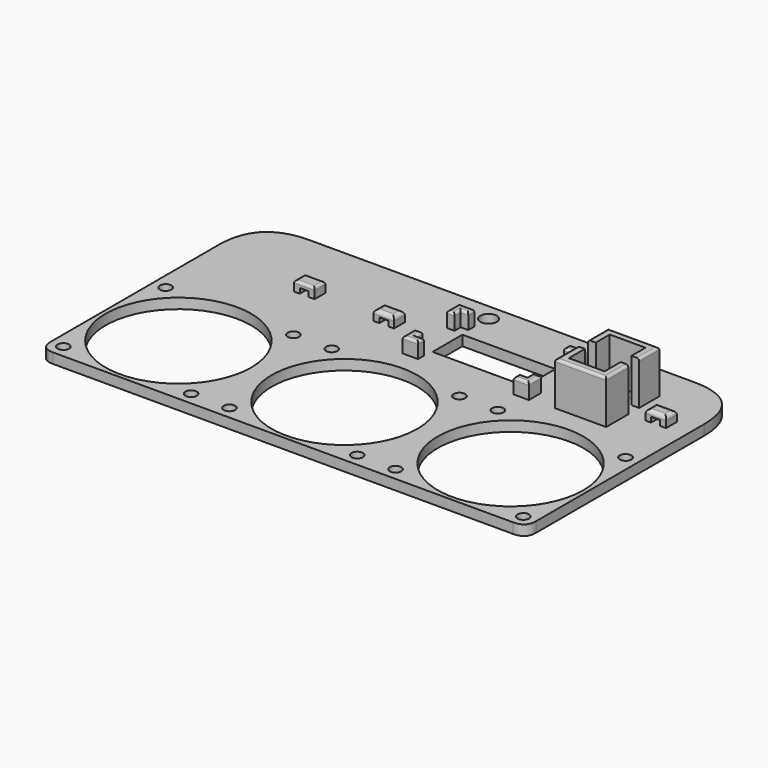
from build123d import *

# Parameters (mm, degrees)
F0_R         = 28.5
F1_DEPTH     = 4
F2_D         = 6.5
F3_D         = 4.5
F5_DEPTH     = 17
F6_DEPTH     = 6
F4_W         = 36.4
F4_H         = 14.6
F7_DEPTH     = 25
F4_W_2       = 7
F4_H_2       = 13
F8_DEPTH     = 25
F9_T1_DEPTH  = 104
F10_T1_DEPTH = 29
F4_W_3       = 8
F4_H_3       = 5.3025707603
F4_H_4       = 5.3
F11_DEPTH    = 4
F12_W        = 3.5351514816
F12_H        = 2
F13_DEPTH    = 25
F14_R        = 1.5
F15_R        = 1
F16_W        = 3.5
F16_H        = 2
F17_DEPTH    = 25
F18_R        = 1.5
F19_W        = 3.5
F19_H        = 2
F20_DEPTH    = 25
F21_R        = 1
F22_R        = 1


# Not quite as in the source:
# - a fillet or chamfer that OpenCascade refuses, or shapes differently, is made with other operations: its cross-section is extruded or revolved along the edge and cut away or added


with BuildPart() as f1:
    # F0 (on Top) → F1 (new body)
    with BuildSketch(Plane.XY):
        Polygon((0, 60), (0, 0), (60, 0), (65, 0), (125, 0), (130, 0), (190, 0), (190, 60), (190, 107), (0, 107), align=None)
        with Locations((30, 30)):
            Circle(F0_R, mode=Mode.SUBTRACT)
        with Locations((95, 30)):
            Circle(F0_R, mode=Mode.SUBTRACT)
        with Locations((160, 30)):
            Circle(F0_R, mode=Mode.SUBTRACT)
    extrude(amount=F1_DEPTH)

    # F2 (through all)
    with Locations(Plane(origin=(0, 0, 0), x_dir=(1, 0, 0), z_dir=(0, 0, -1))):
        with Locations((95, -100.5)):
            Hole(F2_D / 2)

    # F3 (through all)
    with Locations(Plane(origin=(0, 0, 0), x_dir=(1, 0, 0), z_dir=(0, 0, -1))):
        with Locations((5, -55), (55, -55), (5, -5), (55, -5), (70, -55), (70, -5), (120, -5), (120, -55), (135, -55), (135, -5), (185, -5), (185, -55)):
            Hole(F3_D / 2)

    # F4 (on face) → F5 (join)
    with BuildSketch(Plane.XY.offset(4)):
        Polygon((150.7997452021, 83.1751078367), (150.7997452021, 90), (164.7997452021, 90), (164.7997452021, 83.1751078367), (167.7997452021, 83.1751078367), (167.7997452021, 93), (147.7997452021, 93), (147.7997452021, 83.1751078367), align=None)
        Polygon((150.7997452021, 70), (150.7997452021, 77.8725370765), (147.7997452021, 77.8725370765), (147.7997452021, 67), (167.7997452021, 67), (167.7997452021, 77.8725370765), (164.7997452021, 77.8725370765), (164.7997452021, 70), align=None)
    extrude(amount=F5_DEPTH)

    # F4 (on face) → F6 (join)
    with BuildSketch(Plane.XY.offset(4)):
        Polygon((132.2073462009, 93.8), (132.2073462009, 90.8), (135.2073462009, 90.8), (135.2073462009, 87.8), (138.2073462009, 87.8), (138.2073462009, 93.8), align=None)
        Polygon((138.2073462009, 66.2), (138.2073462009, 72.2), (135.2073462009, 72.2), (135.2073462009, 69.2), (132.2073462009, 69.2), (132.2073462009, 66.2), align=None)
        Polygon((88.8073462009, 66.2), (94.8073462009, 66.2), (94.8073462009, 69.2), (91.8073462009, 69.2), (91.8073462009, 72.2), (88.8073462009, 72.2), align=None)
        Polygon((88.8073462009, 87.8), (91.8073462009, 87.8), (91.8073462009, 90.8), (94.8073462009, 90.8), (94.8073462009, 93.8), (88.8073462009, 93.8), align=None)
    extrude(amount=F6_DEPTH)

    # F4 (on face) → F7 (cut)
    with BuildSketch(Plane.XY.offset(4)):
        with Locations((113.5073462009, 80)):
            Rectangle(F4_W, F4_H)
    extrude(amount=-F7_DEPTH, mode=Mode.SUBTRACT)

    # F4 (on face) → F8 (cut)
    with BuildSketch(Plane.XY.offset(4)):
        with Locations((157.7997452021, 80)):
            Rectangle(F4_W_2, F4_H_2)
    extrude(amount=-F8_DEPTH, mode=Mode.SUBTRACT)

    # F9: fillet of radius 20 on 2 edges, made by hand

    # F9_s2 → F9_t1 (cut)
    with BuildSketch(Plane.XY.offset(-50)):
        with BuildLine():
            add(Edge.make_bspline(
                [(0, 87), (0, 107), (20, 107)],
                knots=[0, 0, 0, 1, 1, 1], degree=2, weights=[1, 1, 1]))
            Line((20, 107), (0, 107))
            Line((0, 107), (0, 87))
        make_face()
        with BuildLine():
            add(Edge.make_bspline(
                [(170, 107), (190, 107), (190, 87)],
                knots=[0, 0, 0, 1, 1, 1], degree=2, weights=[1, 1, 1]))
            Line((190, 87), (190, 107))
            Line((190, 107), (170, 107))
        make_face()
    extrude(amount=F9_T1_DEPTH, mode=Mode.SUBTRACT)

    # F10: fillet of radius 5 on 2 edges, made by hand

    # F10_s2 → F10_t1 (cut)
    with BuildSketch(Plane.XY.offset(-12.5)):
        with BuildLine():
            add(Edge.make_bspline(
                [(0, 5), (0, 0), (5, 0)],
                knots=[0, 0, 0, 1, 1, 1], degree=2, weights=[1, 1, 1]))
            Line((5, 0), (0, 0))
            Line((0, 0), (0, 5))
        make_face()
        with BuildLine():
            add(Edge.make_bspline(
                [(185, 0), (190, 0), (190, 5)],
                knots=[0, 0, 0, 1, 1, 1], degree=2, weights=[1, 1, 1]))
            Line((190, 5), (190, 0))
            Line((190, 0), (185, 0))
        make_face()
    extrude(amount=F10_T1_DEPTH, mode=Mode.SUBTRACT)

    # F4 (on face) → F11 (join)
    with BuildSketch(Plane.XY.offset(4)):
        with Locations((178.55278337, 80.5238224566)):
            Rectangle(F4_W_3, F4_H_3)
        with Locations((72.4365121722, 80.0548492312)):
            Rectangle(F4_W_3, F4_H_4)
        with Locations((41.3649373651, 80.0548492312)):
            Rectangle(F4_W_3, F4_H_4)
    extrude(amount=F11_DEPTH)

    # F12 (on face) → F13 (cut)
    with BuildSketch(Plane.XZ.offset(-77.8725370765)):
        with Locations((178.4631460905, 5)):
            Rectangle(F12_W, F12_H)
    extrude(amount=-F13_DEPTH, mode=Mode.SUBTRACT)

    # F14
    f14_edges = [f1.edges().sort_by_distance(p)[0] for p in [
        (174.552783, 80.523822, 8),
        (182.552783, 80.523822, 8),
        (178.552783, 83.175108, 8),
        (178.552783, 77.872537, 8),
    ]]
    fillet(f14_edges, radius=F14_R)

    # F15
    f15_edges = [f1.edges().sort_by_distance(p)[0] for p in [
        (147.799745, 72.436269, 21),
        (157.799745, 67, 21),
        (167.799745, 72.436269, 21),
        (147.799745, 88.087554, 21),
        (157.799745, 93, 21),
        (167.799745, 88.087554, 21),
    ]]
    fillet(f15_edges, radius=F15_R)

    # F16 (on face) → F17 (cut)
    with BuildSketch(Plane.XZ.offset(-77.4048492312)):
        with Locations((72.4831895828, 5)):
            Rectangle(F16_W, F16_H)
    extrude(amount=-F17_DEPTH, mode=Mode.SUBTRACT)

    # F18
    f18_edges = [f1.edges().sort_by_distance(p)[0] for p in [
        (72.436512, 82.704849, 8),
        (68.436512, 80.054849, 8),
        (72.436512, 77.404849, 8),
        (76.436512, 80.054849, 8),
    ]]
    fillet(f18_edges, radius=F18_R)

    # F19 (on face) → F20 (cut)
    with BuildSketch(Plane.XZ.offset(-77.4048492312)):
        with Locations((41.3242319524, 5)):
            Rectangle(F19_W, F19_H)
    extrude(amount=-F20_DEPTH, mode=Mode.SUBTRACT)

    # F21
    f21_edges = [f1.edges().sort_by_distance(p)[0] for p in [
        (41.364937, 77.404849, 8),
        (45.364937, 80.054849, 8),
        (41.364937, 82.704849, 8),
        (37.364937, 80.054849, 8),
    ]]
    fillet(f21_edges, radius=F21_R)

    # F22
    f22_edges = [f1.edges().sort_by_distance(p)[0] for p in [
        (90.307346, 87.8, 10),
        (91.807346, 89.3, 10),
        (93.307346, 90.8, 10),
        (94.807346, 92.3, 10),
        (91.807346, 93.8, 10),
        (88.807346, 90.8, 10),
        (132.207346, 92.3, 10),
        (133.707346, 90.8, 10),
        (135.207346, 89.3, 10),
        (136.707346, 87.8, 10),
        (138.207346, 90.8, 10),
        (135.207346, 93.8, 10),
        (138.207346, 69.2, 10),
        (136.707346, 72.2, 10),
        (135.207346, 70.7, 10),
        (133.707346, 69.2, 10),
        (132.207346, 67.7, 10),
        (135.207346, 66.2, 10),
        (91.807346, 66.2, 10),
        (94.807346, 67.7, 10),
        (93.307346, 69.2, 10),
        (91.807346, 70.7, 10),
        (90.307346, 72.2, 10),
        (88.807346, 69.2, 10),
    ]]
    fillet(f22_edges, radius=F22_R)


solid = f1.part
